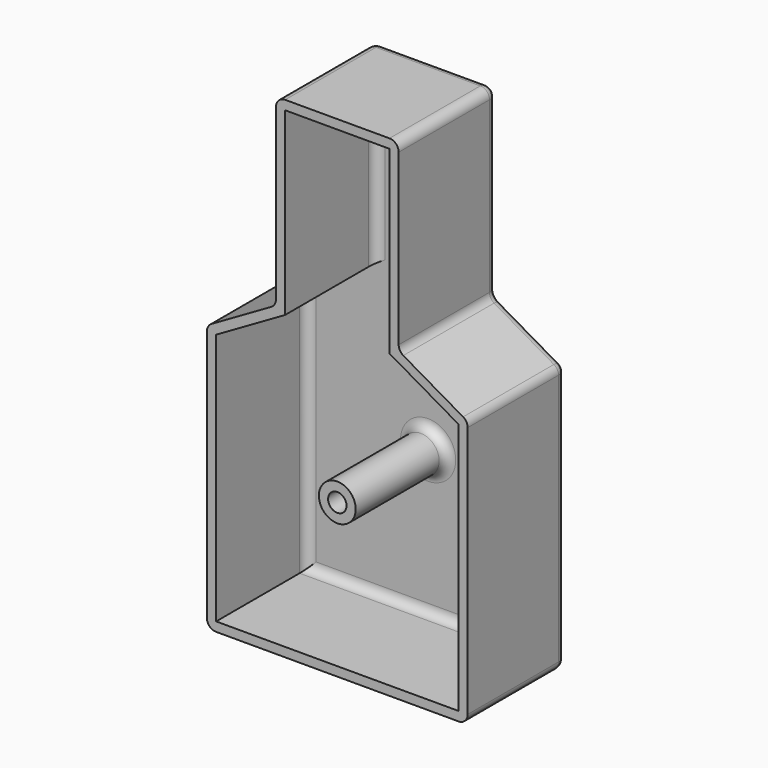
from build123d import *

# Parameters (mm, degrees)
F1_R     = 3
F2_DEPTH = 40
F3_T     = -3
F4_R     = 3


with BuildPart() as f2:
    # F1 (on Front) → F2 (new body)
    with BuildSketch(Plane.XZ):
        Polygon((42.5, 37.0096189432), (20, 50), (20, 110), (-20, 110), (-20, 50), (-42.5, 37.0096189432), (-42.5, -50), (42.5, -50), align=None)
        Circle(F1_R, mode=Mode.SUBTRACT)
    extrude(amount=F2_DEPTH)

    # F3
    f3_openings = [f2.faces().sort_by_distance(p)[0] for p in [
        (0, -40, 16.88666),
    ]]
    offset(amount=F3_T, openings=f3_openings, kind=Kind.INTERSECTION)

    # F4
    f4_edges = [f2.edges().sort_by_distance(p)[0] for p in [
        (39.5, -3, -5.861216),
        (0, -3, -47),
        (-39.5, -3, -5.861216),
        (17, -3, 77.633975),
        (0, -3, 107),
        (-17, -3, 77.633975),
        (-20, -20, 110),
        (20, -20, 110),
        (42.5, -20, -50),
        (-42.5, -20, -50),
        (0, 0, 110),
        (20, 0, 80),
        (-42.5, 0, -6.495191),
        (-20, 0, 80),
        (0, 0, -50),
        (42.5, 0, -6.495191),
        (-6, -3, 0),
        (42.5, -20, 37.009619),
        (20, -20, 50),
        (31.25, 0, 43.504809),
        (-20, -20, 50),
        (-42.5, -20, 37.009619),
        (-31.25, 0, 43.504809),
    ]]
    fillet(f4_edges, radius=F4_R)


solid = f2.part
